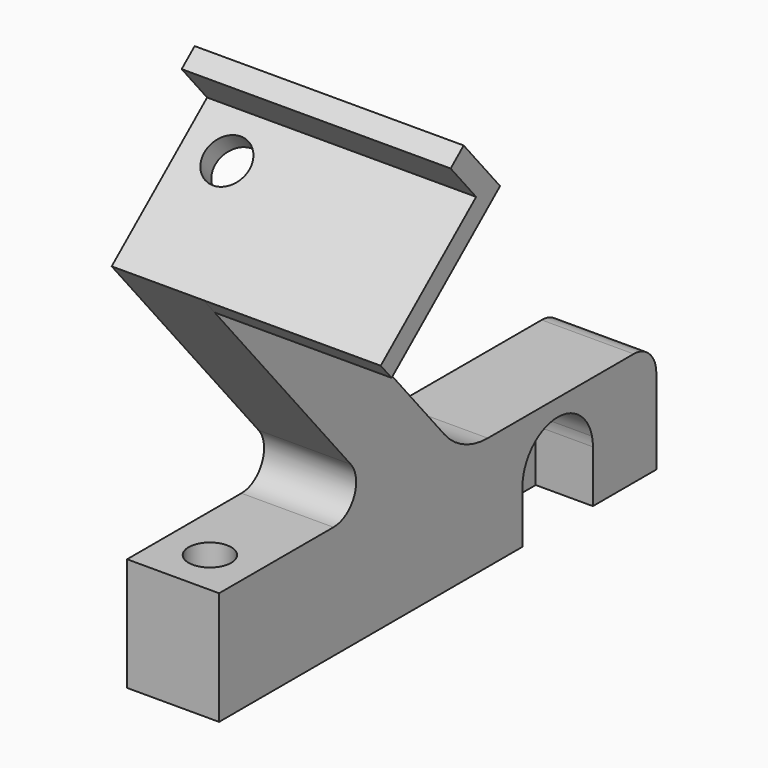
from build123d import *

# Parameters (mm, degrees)
F0_R      = 4.415
F0_W      = 3.025
F0_H      = 16
F0_W_2    = 7.0735459991
F1_DEPTH  = 13
F3_DEPTH  = 8.075
F4_R      = 10
F5_R      = 3
F6_DEPTH  = 25
F7_R      = 3.2
F8_DEPTH  = 11.1
F10_DEPTH = 25


# Not quite as in the source:
# - ends of sketch curves that miss each other by under 0.0002 mm in the source are joined


with BuildPart() as f1:
    # F0 (on Right) → F1 (new body)
    with BuildSketch(Plane.YZ):
        with BuildLine():
            Line((-11.2, 0), (0, 0))
            Line((0, 0), (0, 12))
            ThreePointArc((0, 12), (-1.1715728753, 14.8284271247), (-4, 16))
            Line((-4, 16), (-34.4146185314, 16))
            Line((-34.4146185314, 16), (-69.7679370642, 58.1324443715))
            Line((-69.7679370642, 58.1324443715), (-58.8383850945, 67.3034273983))
            Line((-58.8383850945, 67.3034273983), (-65.2662611913, 74.9638718294))
            Line((-65.2662611913, 74.9638718294), (-67.5643945207, 73.0355090004))
            Line((-67.5643945207, 73.0355090004), (-63.0648812529, 67.6731978986))
            Line((-63.0648812529, 67.6731978986), (-79.9178590015, 53.5318704855))
            Line((-79.9178590015, 53.5318704855), (-53.9387302293, 22.5711504387))
            ThreePointArc((-53.9387302293, 22.5711504387), (-53.3776768537, 18.309526953), (-57.0029080018, 16))
            Line((-57.0029080018, 16), (-67.1014540009, 16))
            Line((-67.1014540009, 16), (-67.1014540009, 0))
            Line((-67.1014540009, 0), (-64.0764540009, 0))
            Line((-64.0764540009, 0), (-23.65, 0))
            Line((-23.65, 0), (-23.65, 7.375))
            ThreePointArc((-23.65, 7.375), (-21.8267397129, 11.7767397129), (-17.425, 13.6))
            ThreePointArc((-17.425, 13.6), (-13.0232602871, 11.7767397129), (-11.2, 7.375))
            Line((-11.2, 7.375), (-11.2, 0))
        make_face()
        with BuildLine():
            Line((-23.65, 0), (-11.2, 0))
            Line((-11.2, 0), (-11.2, 7.375))
            ThreePointArc((-11.2, 7.375), (-13.0232602871, 11.7767397129), (-17.425, 13.6))
            ThreePointArc((-17.425, 13.6), (-21.8267397129, 11.7767397129), (-23.65, 7.375))
            Line((-23.65, 7.375), (-23.65, 0))
        make_face()
        with Locations((-17.425, 7.375)):
            Circle(F0_R, mode=Mode.SUBTRACT)
        with Locations((-68.6139540009, 8)):
            Rectangle(F0_W, F0_H)
        with Locations((-73.6632270005, 8)):
            Rectangle(F0_W_2, F0_H)
    extrude(amount=-F1_DEPTH)

    # F2 (on face) → F3 (cut)
    with BuildSketch(Plane.YZ):
        with BuildLine():
            Line((-17.425, 0), (-11.2, 0))
            Line((-11.2, 0), (-11.2, 7.3750006942))
            ThreePointArc((-11.2, 7.3750006942), (-11.2387169647, 8.068201392), (-11.3543862514, 8.7527792377))
            ThreePointArc((-11.3543862514, 8.7527792377), (-18.1182010341, 13.5612829976), (-23.65, 7.375))
            Line((-23.65, 7.375), (-23.65, 0))
            Line((-23.65, 0), (-17.425, 0))
        make_face()
        with BuildLine():
            ThreePointArc((-13.01, 7.375), (-14.3031235611, 4.2531235611), (-17.425, 2.96))
            ThreePointArc((-17.425, 2.96), (-20.5468764389, 10.4968764389), (-13.01, 7.375))
        make_face(mode=Mode.SUBTRACT)
    extrude(amount=-F3_DEPTH, mode=Mode.SUBTRACT)

    # F4
    f4_edges = [f1.edges().sort_by_distance(p)[0] for p in [
        (-6.5, -34.414619, 16),
    ]]
    fillet(f4_edges, radius=F4_R)

    # F5 (on face) → F6 (cut)
    with BuildSketch(Plane.XY.offset(16)):
        with Locations((-6.5, -70.7)):
            Circle(F5_R)
    extrude(amount=-F6_DEPTH, mode=Mode.SUBTRACT)

    # F7 (on face) → F8 (cut)
    with BuildSketch(Plane(origin=(0, -59.3794347551, 70.7656546956), x_dir=(1, 0, 0), z_dir=(0, -0.6427876097, 0.7660444431))):
        with Locations((-6.5, -10.8610087227)):
            Circle(F7_R)
    extrude(amount=-F8_DEPTH, mode=Mode.SUBTRACT)

    # F9 (on face) → F10 (join)
    with BuildSketch(Plane.YZ):
        Polygon((-77.9894961724, 51.2337371561), (-58.8383850945, 67.3034273983), (-65.2662611913, 74.9638718294), (-67.5643945207, 73.0355090004), (-63.0648812529, 67.6731978986), (-79.9178590015, 53.5318704855), align=None)
    extrude(amount=F10_DEPTH)


solid = f1.part
